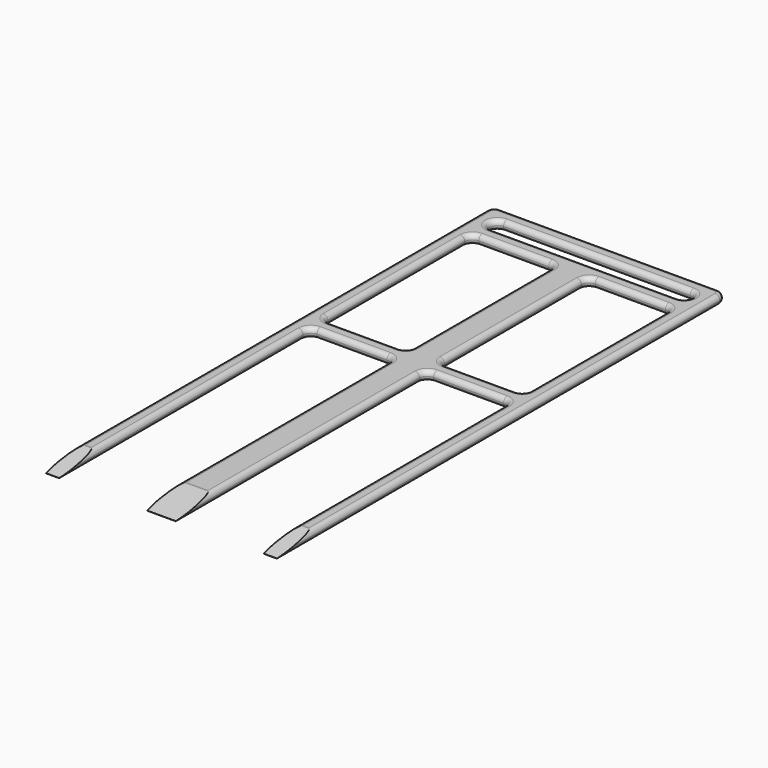
from build123d import *

# Parameters (mm, degrees)
F1_DEPTH     = 3
F2_SIZE2     = 14.178204549
F2_SIZE      = 2.5
F2_2_SIZE2   = 14.178204549
F2_2_SIZE    = 2.5
F2_3_SIZE2   = 14.178204549
F2_3_SIZE    = 2.5
F3_T1_DEPTH  = 174.571795451
F3_T3_DEPTH  = 5.6561649764
F3_T5_DEPTH  = 94.571795451
F3_T7_DEPTH  = 70
F3_T9_DEPTH  = 22.5
F3_T11_DEPTH = 5.6561649764
F3_T13_DEPTH = 10.6561649764
F3_T15_DEPTH = 22.5
F3_T17_DEPTH = 55
F3_T19_DEPTH = 60
F3_T21_DEPTH = 181.25
F3_T23_DEPTH = 10.5901699437
F3_T25_DEPTH = 101.25
F3_T27_DEPTH = 15.5901699437
F3_T29_DEPTH = 10.5901699437
F3_T32_ANGLE = 90
F3_T34_ANGLE = 90
F3_T36_ANGLE = 90
F3_T38_ANGLE = 90
F3_T40_ANGLE = 90
F3_T42_ANGLE = 90
F3_T44_ANGLE = 90
F3_T46_ANGLE = 90
F3_T48_ANGLE = 90
F3_T50_ANGLE = 90
F3_T52_ANGLE = 180
F3_T54_ANGLE = 180
F3_T56_ANGLE = 90
F3_T58_ANGLE = 90
F3_T60_ANGLE = 90
F3_T62_ANGLE = 90
F3_T64_ANGLE = 90
F3_T66_ANGLE = 90
F3_T68_ANGLE = 90
F3_T70_ANGLE = 90
F3_T72_ANGLE = 90
F3_T74_ANGLE = 90
F3_T76_ANGLE = 90
F3_T78_ANGLE = 90
F3_T80_ANGLE = 90
F3_T82_ANGLE = 90
F3_T84_ANGLE = 180
F3_T86_ANGLE = 180
F3_T88_ANGLE = 90
F3_T90_ANGLE = 90
F3_T92_ANGLE = 90
F3_T94_ANGLE = 90


# Not quite as in the source:
# - a fillet or chamfer that OpenCascade refuses, or shapes differently, is made with other operations: its cross-section is extruded or revolved along the edge and cut away or added


with BuildPart() as f1:
    # F0 (on Top) → F1 (new body)
    with BuildSketch(Plane.XY):
        with BuildLine():
            ThreePointArc((37.5, 87.5), (36.767766953, 89.267766953), (35, 90))
            Line((35, 90), (-35, 90))
            ThreePointArc((-35, 90), (-36.767766953, 89.267766953), (-37.5, 87.5))
            Line((-37.5, 87.5), (-37.5, -90))
            Line((-37.5, -90), (-32.5, -90))
            Line((-32.5, -90), (-32.5, 7.5))
            ThreePointArc((-32.5, 7.5), (-31.767766953, 9.267766953), (-30, 10))
            Line((-30, 10), (-7.5, 10))
            ThreePointArc((-7.5, 10), (-5.732233047, 9.267766953), (-5, 7.5))
            Line((-5, 7.5), (-5, -90))
            Line((-5, -90), (5, -90))
            Line((5, -90), (5, 7.5))
            ThreePointArc((5, 7.5), (5.732233047, 9.267766953), (7.5, 10))
            Line((7.5, 10), (30, 10))
            ThreePointArc((30, 10), (31.767766953, 9.267766953), (32.5, 7.5))
            Line((32.5, 7.5), (32.5, -90))
            Line((32.5, -90), (37.5, -90))
            Line((37.5, -90), (37.5, 87.5))
        make_face()
        with BuildLine():
            ThreePointArc((-5, 17.5), (-5.732233047, 15.732233047), (-7.5, 15))
            Line((-7.5, 15), (-30, 15))
            ThreePointArc((-30, 15), (-31.767766953, 15.732233047), (-32.5, 17.5))
            Line((-32.5, 17.5), (-32.5, 72.5))
            ThreePointArc((-32.5, 72.5), (-31.767766953, 74.267766953), (-30, 75))
            Line((-30, 75), (-7.5, 75))
            ThreePointArc((-7.5, 75), (-5.732233047, 74.267766953), (-5, 72.5))
            Line((-5, 72.5), (-5, 17.5))
        make_face(mode=Mode.SUBTRACT)
        with BuildLine():
            ThreePointArc((32.5, 82.5), (31.767766953, 80.732233047), (30, 80))
            Line((30, 80), (-30, 80))
            ThreePointArc((-30, 80), (-31.767766953, 80.732233047), (-32.5, 82.5))
            ThreePointArc((-32.5, 82.5), (-31.767766953, 84.267766953), (-30, 85))
            Line((-30, 85), (30, 85))
            ThreePointArc((30, 85), (31.767766953, 84.267766953), (32.5, 82.5))
        make_face(mode=Mode.SUBTRACT)
        with BuildLine():
            ThreePointArc((32.5, 17.5), (31.767766953, 15.732233047), (30, 15))
            Line((30, 15), (7.5, 15))
            ThreePointArc((7.5, 15), (5.732233047, 15.732233047), (5, 17.5))
            Line((5, 17.5), (5, 72.5))
            ThreePointArc((5, 72.5), (5.732233047, 74.267766953), (7.5, 75))
            Line((7.5, 75), (30, 75))
            ThreePointArc((30, 75), (31.767766953, 74.267766953), (32.5, 72.5))
            Line((32.5, 72.5), (32.5, 17.5))
        make_face(mode=Mode.SUBTRACT)
    extrude(amount=F1_DEPTH)

    # F2
    f2_edges = [f1.edges().sort_by_distance(p)[0] for p in [
        (0, -90, 3),
    ]]
    f2_side = f1.faces().sort_by_distance((0, -90, 1.5))[0]
    chamfer(f2_edges, length=F2_SIZE, length2=F2_SIZE2, reference=f2_side)

    # F2#2
    f2_2_edges = [f1.edges().sort_by_distance(p)[0] for p in [
        (35, -90, 3),
    ]]
    f2_2_side = f1.faces().sort_by_distance((35, -90, 1.5))[0]
    chamfer(f2_2_edges, length=F2_2_SIZE, length2=F2_2_SIZE2, reference=f2_2_side)

    # F2#3
    f2_3_edges = [f1.edges().sort_by_distance(p)[0] for p in [
        (-35, -90, 3),
    ]]
    f2_3_side = f1.faces().sort_by_distance((-35, -90, 1.5))[0]
    chamfer(f2_3_edges, length=F2_3_SIZE, length2=F2_3_SIZE2, reference=f2_3_side)

    # F3: fillet of radius 1.5 on 76 edges, made by hand

    # F3_s2 → F3_t1 (cut)
    with BuildSketch(Plane.XZ.offset(-87.5)):
        with BuildLine():
            ThreePointArc((-36, 3), (-37.0606601718, 2.5606601718), (-37.5, 1.5))
            Line((-37.5, 1.5), (-37.53, 1.5))
            Line((-37.53, 1.5), (-37.53, 3.03))
            Line((-37.53, 3.03), (-36, 3.03))
            Line((-36, 3.03), (-36, 3))
        make_face()
        with BuildLine():
            ThreePointArc((36, 3), (37.0606601718, 2.5606601718), (37.5, 1.5))
            Line((37.5, 1.5), (37.53, 1.5))
            Line((37.53, 1.5), (37.53, 3.03))
            Line((37.53, 3.03), (36, 3.03))
            Line((36, 3.03), (36, 3))
        make_face()
    extrude(amount=F3_T1_DEPTH, mode=Mode.SUBTRACT)

    # F3_s4 → F3_t3 (cut)
    with BuildSketch(Plane.YZ.offset(-37.8280824882)):
        with BuildLine():
            ThreePointArc((-75.6905624557, 3), (-75.8212960698, 2.9942920471), (-75.9510347222, 2.9772116295))
            Line((-75.9510347222, 2.9772116295), (-75.9562441675, 3.0067558621))
            Line((-75.9562441675, 3.0067558621), (-75.8244201109, 3.03))
            Line((-75.8244201109, 3.03), (-75.6905624557, 3.03))
            Line((-75.6905624557, 3.03), (-75.6905624557, 3))
        make_face()
    extrude(amount=F3_T3_DEPTH, mode=Mode.SUBTRACT)

    # F3_s6 → F3_t5 (cut)
    with BuildSketch(Plane.XZ.offset(-7.5)):
        with BuildLine():
            ThreePointArc((-34, 3), (-32.9393398282, 2.5606601718), (-32.5, 1.5))
            Line((-32.5, 1.5), (-32.47, 1.5))
            Line((-32.47, 1.5), (-32.47, 3.03))
            Line((-32.47, 3.03), (-34, 3.03))
            Line((-34, 3.03), (-34, 3))
        make_face()
        with BuildLine():
            ThreePointArc((-3.5, 3), (-4.5606601718, 2.5606601718), (-5, 1.5))
            Line((-5, 1.5), (-5.03, 1.5))
            Line((-5.03, 1.5), (-5.03, 3.03))
            Line((-5.03, 3.03), (-3.5, 3.03))
            Line((-3.5, 3.03), (-3.5, 3))
        make_face()
        with BuildLine():
            ThreePointArc((34, 3), (32.9393398282, 2.5606601718), (32.5, 1.5))
            Line((32.5, 1.5), (32.47, 1.5))
            Line((32.47, 1.5), (32.47, 3.03))
            Line((32.47, 3.03), (34, 3.03))
            Line((34, 3.03), (34, 3))
        make_face()
        with BuildLine():
            ThreePointArc((3.5, 3), (4.5606601718, 2.5606601718), (5, 1.5))
            Line((5, 1.5), (5.03, 1.5))
            Line((5.03, 1.5), (5.03, 3.03))
            Line((5.03, 3.03), (3.5, 3.03))
            Line((3.5, 3.03), (3.5, 3))
        make_face()
    extrude(amount=F3_T5_DEPTH, mode=Mode.SUBTRACT)

    # F3_s8 → F3_t7 (cut)
    with BuildSketch(Plane.YZ.offset(-35)):
        with BuildLine():
            ThreePointArc((88.5, 3), (89.5606601718, 2.5606601718), (90, 1.5))
            Line((90, 1.5), (90.03, 1.5))
            Line((90.03, 1.5), (90.03, 3.03))
            Line((90.03, 3.03), (88.5, 3.03))
            Line((88.5, 3.03), (88.5, 3))
        make_face()
        with BuildLine():
            ThreePointArc((90, 1.5), (89.5606601718, 0.4393398282), (88.5, 0))
            Line((88.5, 0), (88.5, -0.03))
            Line((88.5, -0.03), (90.03, -0.03))
            Line((90.03, -0.03), (90.03, 1.5))
            Line((90.03, 1.5), (90, 1.5))
        make_face()
    extrude(amount=F3_T7_DEPTH, mode=Mode.SUBTRACT)

    # F3_s10 → F3_t9 (cut)
    with BuildSketch(Plane.YZ.offset(-30)):
        with BuildLine():
            ThreePointArc((11.5, 3), (10.4393398282, 2.5606601718), (10, 1.5))
            Line((10, 1.5), (9.97, 1.5))
            Line((9.97, 1.5), (9.97, 3.03))
            Line((9.97, 3.03), (11.5, 3.03))
            Line((11.5, 3.03), (11.5, 3))
        make_face()
        with BuildLine():
            ThreePointArc((13.5, 3), (14.5606601718, 2.5606601718), (15, 1.5))
            Line((15, 1.5), (15.03, 1.5))
            Line((15.03, 1.5), (15.03, 3.03))
            Line((15.03, 3.03), (13.5, 3.03))
            Line((13.5, 3.03), (13.5, 3))
        make_face()
        with BuildLine():
            ThreePointArc((76.5, 3), (75.4393398282, 2.5606601718), (75, 1.5))
            Line((75, 1.5), (74.97, 1.5))
            Line((74.97, 1.5), (74.97, 3.03))
            Line((74.97, 3.03), (76.5, 3.03))
            Line((76.5, 3.03), (76.5, 3))
        make_face()
        with BuildLine():
            ThreePointArc((10, 1.5), (10.4393398282, 0.4393398282), (11.5, 0))
            Line((11.5, 0), (11.5, -0.03))
            Line((11.5, -0.03), (9.97, -0.03))
            Line((9.97, -0.03), (9.97, 1.5))
            Line((9.97, 1.5), (10, 1.5))
        make_face()
        with BuildLine():
            ThreePointArc((15, 1.5), (14.5606601718, 0.4393398282), (13.5, 0))
            Line((13.5, 0), (13.5, -0.03))
            Line((13.5, -0.03), (15.03, -0.03))
            Line((15.03, -0.03), (15.03, 1.5))
            Line((15.03, 1.5), (15, 1.5))
        make_face()
        with BuildLine():
            ThreePointArc((75, 1.5), (75.4393398282, 0.4393398282), (76.5, 0))
            Line((76.5, 0), (76.5, -0.03))
            Line((76.5, -0.03), (74.97, -0.03))
            Line((74.97, -0.03), (74.97, 1.5))
            Line((74.97, 1.5), (75, 1.5))
        make_face()
    extrude(amount=F3_T9_DEPTH, mode=Mode.SUBTRACT)

    # F3_s12 → F3_t11 (cut)
    with BuildSketch(Plane.YZ.offset(32.1719175118)):
        with BuildLine():
            ThreePointArc((-75.6905624557, 3), (-75.8212960698, 2.9942920471), (-75.9510347222, 2.9772116295))
            Line((-75.9510347222, 2.9772116295), (-75.9562441675, 3.0067558621))
            Line((-75.9562441675, 3.0067558621), (-75.8244201109, 3.03))
            Line((-75.8244201109, 3.03), (-75.6905624557, 3.03))
            Line((-75.6905624557, 3.03), (-75.6905624557, 3))
        make_face()
    extrude(amount=F3_T11_DEPTH, mode=Mode.SUBTRACT)

    # F3_s14 → F3_t13 (cut)
    with BuildSketch(Plane.YZ.offset(-5.3280824882)):
        with BuildLine():
            ThreePointArc((-75.6905624557, 3), (-75.8212960698, 2.9942920471), (-75.9510347222, 2.9772116295))
            Line((-75.9510347222, 2.9772116295), (-75.9562441675, 3.0067558621))
            Line((-75.9562441675, 3.0067558621), (-75.8244201109, 3.03))
            Line((-75.8244201109, 3.03), (-75.6905624557, 3.03))
            Line((-75.6905624557, 3.03), (-75.6905624557, 3))
        make_face()
    extrude(amount=F3_T13_DEPTH, mode=Mode.SUBTRACT)

    # F3_s16 → F3_t15 (cut)
    with BuildSketch(Plane.YZ.offset(7.5)):
        with BuildLine():
            ThreePointArc((11.5, 3), (10.4393398282, 2.5606601718), (10, 1.5))
            Line((10, 1.5), (9.97, 1.5))
            Line((9.97, 1.5), (9.97, 3.03))
            Line((9.97, 3.03), (11.5, 3.03))
            Line((11.5, 3.03), (11.5, 3))
        make_face()
        with BuildLine():
            ThreePointArc((13.5, 3), (14.5606601718, 2.5606601718), (15, 1.5))
            Line((15, 1.5), (15.03, 1.5))
            Line((15.03, 1.5), (15.03, 3.03))
            Line((15.03, 3.03), (13.5, 3.03))
            Line((13.5, 3.03), (13.5, 3))
        make_face()
        with BuildLine():
            ThreePointArc((76.5, 3), (75.4393398282, 2.5606601718), (75, 1.5))
            Line((75, 1.5), (74.97, 1.5))
            Line((74.97, 1.5), (74.97, 3.03))
            Line((74.97, 3.03), (76.5, 3.03))
            Line((76.5, 3.03), (76.5, 3))
        make_face()
        with BuildLine():
            ThreePointArc((10, 1.5), (10.4393398282, 0.4393398282), (11.5, 0))
            Line((11.5, 0), (11.5, -0.03))
            Line((11.5, -0.03), (9.97, -0.03))
            Line((9.97, -0.03), (9.97, 1.5))
            Line((9.97, 1.5), (10, 1.5))
        make_face()
        with BuildLine():
            ThreePointArc((15, 1.5), (14.5606601718, 0.4393398282), (13.5, 0))
            Line((13.5, 0), (13.5, -0.03))
            Line((13.5, -0.03), (15.03, -0.03))
            Line((15.03, -0.03), (15.03, 1.5))
            Line((15.03, 1.5), (15, 1.5))
        make_face()
        with BuildLine():
            ThreePointArc((75, 1.5), (75.4393398282, 0.4393398282), (76.5, 0))
            Line((76.5, 0), (76.5, -0.03))
            Line((76.5, -0.03), (74.97, -0.03))
            Line((74.97, -0.03), (74.97, 1.5))
            Line((74.97, 1.5), (75, 1.5))
        make_face()
    extrude(amount=F3_T15_DEPTH, mode=Mode.SUBTRACT)

    # F3_s18 → F3_t17 (cut)
    with BuildSketch(Plane.XZ.offset(-72.5)):
        with BuildLine():
            ThreePointArc((-34, 3), (-32.9393398282, 2.5606601718), (-32.5, 1.5))
            Line((-32.5, 1.5), (-32.47, 1.5))
            Line((-32.47, 1.5), (-32.47, 3.03))
            Line((-32.47, 3.03), (-34, 3.03))
            Line((-34, 3.03), (-34, 3))
        make_face()
        with BuildLine():
            ThreePointArc((-3.5, 3), (-4.5606601718, 2.5606601718), (-5, 1.5))
            Line((-5, 1.5), (-5.03, 1.5))
            Line((-5.03, 1.5), (-5.03, 3.03))
            Line((-5.03, 3.03), (-3.5, 3.03))
            Line((-3.5, 3.03), (-3.5, 3))
        make_face()
        with BuildLine():
            ThreePointArc((34, 3), (32.9393398282, 2.5606601718), (32.5, 1.5))
            Line((32.5, 1.5), (32.47, 1.5))
            Line((32.47, 1.5), (32.47, 3.03))
            Line((32.47, 3.03), (34, 3.03))
            Line((34, 3.03), (34, 3))
        make_face()
        with BuildLine():
            ThreePointArc((3.5, 3), (4.5606601718, 2.5606601718), (5, 1.5))
            Line((5, 1.5), (5.03, 1.5))
            Line((5.03, 1.5), (5.03, 3.03))
            Line((5.03, 3.03), (3.5, 3.03))
            Line((3.5, 3.03), (3.5, 3))
        make_face()
        with BuildLine():
            ThreePointArc((-32.5, 1.5), (-32.9393398282, 0.4393398282), (-34, 0))
            Line((-34, 0), (-34, -0.03))
            Line((-34, -0.03), (-32.47, -0.03))
            Line((-32.47, -0.03), (-32.47, 1.5))
            Line((-32.47, 1.5), (-32.5, 1.5))
        make_face()
        with BuildLine():
            ThreePointArc((-5, 1.5), (-4.5606601718, 0.4393398282), (-3.5, 0))
            Line((-3.5, 0), (-3.5, -0.03))
            Line((-3.5, -0.03), (-5.03, -0.03))
            Line((-5.03, -0.03), (-5.03, 1.5))
            Line((-5.03, 1.5), (-5, 1.5))
        make_face()
        with BuildLine():
            ThreePointArc((32.5, 1.5), (32.9393398282, 0.4393398282), (34, 0))
            Line((34, 0), (34, -0.03))
            Line((34, -0.03), (32.47, -0.03))
            Line((32.47, -0.03), (32.47, 1.5))
            Line((32.47, 1.5), (32.5, 1.5))
        make_face()
        with BuildLine():
            ThreePointArc((5, 1.5), (4.5606601718, 0.4393398282), (3.5, 0))
            Line((3.5, 0), (3.5, -0.03))
            Line((3.5, -0.03), (5.03, -0.03))
            Line((5.03, -0.03), (5.03, 1.5))
            Line((5.03, 1.5), (5, 1.5))
        make_face()
    extrude(amount=F3_T17_DEPTH, mode=Mode.SUBTRACT)

    # F3_s20 → F3_t19 (cut)
    with BuildSketch(Plane.YZ.offset(-30)):
        with BuildLine():
            ThreePointArc((78.5, 3), (79.5606601718, 2.5606601718), (80, 1.5))
            Line((80, 1.5), (80.03, 1.5))
            Line((80.03, 1.5), (80.03, 3.03))
            Line((80.03, 3.03), (78.5, 3.03))
            Line((78.5, 3.03), (78.5, 3))
        make_face()
        with BuildLine():
            ThreePointArc((86.5, 3), (85.4393398282, 2.5606601718), (85, 1.5))
            Line((85, 1.5), (84.97, 1.5))
            Line((84.97, 1.5), (84.97, 3.03))
            Line((84.97, 3.03), (86.5, 3.03))
            Line((86.5, 3.03), (86.5, 3))
        make_face()
        with BuildLine():
            ThreePointArc((80, 1.5), (79.5606601718, 0.4393398282), (78.5, 0))
            Line((78.5, 0), (78.5, -0.03))
            Line((78.5, -0.03), (80.03, -0.03))
            Line((80.03, -0.03), (80.03, 1.5))
            Line((80.03, 1.5), (80, 1.5))
        make_face()
        with BuildLine():
            ThreePointArc((85, 1.5), (85.4393398282, 0.4393398282), (86.5, 0))
            Line((86.5, 0), (86.5, -0.03))
            Line((86.5, -0.03), (84.97, -0.03))
            Line((84.97, -0.03), (84.97, 1.5))
            Line((84.97, 1.5), (85, 1.5))
        make_face()
    extrude(amount=F3_T19_DEPTH, mode=Mode.SUBTRACT)

    # F3_s22 → F3_t21 (cut)
    with BuildSketch(Plane.XZ.offset(-87.5)):
        with BuildLine():
            ThreePointArc((-37.5, 1.5), (-37.0606601718, 0.4393398282), (-36, 0))
            Line((-36, 0), (-36, -0.03))
            Line((-36, -0.03), (-37.53, -0.03))
            Line((-37.53, -0.03), (-37.53, 1.5))
            Line((-37.53, 1.5), (-37.5, 1.5))
        make_face()
        with BuildLine():
            ThreePointArc((37.5, 1.5), (37.0606601718, 0.4393398282), (36, 0))
            Line((36, 0), (36, -0.03))
            Line((36, -0.03), (37.53, -0.03))
            Line((37.53, -0.03), (37.53, 1.5))
            Line((37.53, 1.5), (37.5, 1.5))
        make_face()
    extrude(amount=F3_T21_DEPTH, mode=Mode.SUBTRACT)

    # F3_s24 → F3_t23 (cut)
    with BuildSketch(Plane.YZ.offset(-40.2950849719)):
        with BuildLine():
            ThreePointArc((-90, 0.5), (-89.4943384469, 0.1306936062), (-88.8819660113, 0))
            Line((-88.8819660113, 0), (-88.8819660113, -0.03))
            Line((-88.8819660113, -0.03), (-90, -0.03))
            Line((-90, -0.03), (-90.03, 0))
            ThreePointArc((-90.03, 0), (-90.03, 0.25), (-90.0223606798, 0.48))
            Line((-90.0223606798, 0.48), (-90, 0.5))
        make_face()
    extrude(amount=F3_T23_DEPTH, mode=Mode.SUBTRACT)

    # F3_s26 → F3_t25 (cut)
    with BuildSketch(Plane.XZ.offset(-7.5)):
        with BuildLine():
            ThreePointArc((-32.5, 1.5), (-32.9393398282, 0.4393398282), (-34, 0))
            Line((-34, 0), (-34, -0.03))
            Line((-34, -0.03), (-32.47, -0.03))
            Line((-32.47, -0.03), (-32.47, 1.5))
            Line((-32.47, 1.5), (-32.5, 1.5))
        make_face()
        with BuildLine():
            ThreePointArc((-5, 1.5), (-4.5606601718, 0.4393398282), (-3.5, 0))
            Line((-3.5, 0), (-3.5, -0.03))
            Line((-3.5, -0.03), (-5.03, -0.03))
            Line((-5.03, -0.03), (-5.03, 1.5))
            Line((-5.03, 1.5), (-5, 1.5))
        make_face()
        with BuildLine():
            ThreePointArc((5, 1.5), (4.5606601718, 0.4393398282), (3.5, 0))
            Line((3.5, 0), (3.5, -0.03))
            Line((3.5, -0.03), (5.03, -0.03))
            Line((5.03, -0.03), (5.03, 1.5))
            Line((5.03, 1.5), (5, 1.5))
        make_face()
        with BuildLine():
            ThreePointArc((32.5, 1.5), (32.9393398282, 0.4393398282), (34, 0))
            Line((34, 0), (34, -0.03))
            Line((34, -0.03), (32.47, -0.03))
            Line((32.47, -0.03), (32.47, 1.5))
            Line((32.47, 1.5), (32.5, 1.5))
        make_face()
    extrude(amount=F3_T25_DEPTH, mode=Mode.SUBTRACT)

    # F3_s28 → F3_t27 (cut)
    with BuildSketch(Plane.YZ.offset(-7.7950849719)):
        with BuildLine():
            ThreePointArc((-88.8819660113, 0), (-89.4943384469, 0.1306936062), (-90, 0.5))
            Line((-90, 0.5), (-90.0223606798, 0.48))
            ThreePointArc((-90.0223606798, 0.48), (-90.03, 0.25), (-90.03, 0))
            Line((-90.03, 0), (-90, -0.03))
            Line((-90, -0.03), (-88.8819660113, -0.03))
            Line((-88.8819660113, -0.03), (-88.8819660113, 0))
        make_face()
    extrude(amount=F3_T27_DEPTH, mode=Mode.SUBTRACT)

    # F3_s30 → F3_t29 (cut)
    with BuildSketch(Plane.YZ.offset(29.7049150281)):
        with BuildLine():
            ThreePointArc((-88.8819660113, 0), (-89.4943384469, 0.1306936062), (-90, 0.5))
            Line((-90, 0.5), (-90.0223606798, 0.48))
            ThreePointArc((-90.0223606798, 0.48), (-90.03, 0.25), (-90.03, 0))
            Line((-90.03, 0), (-90, -0.03))
            Line((-90, -0.03), (-88.8819660113, -0.03))
            Line((-88.8819660113, -0.03), (-88.8819660113, 0))
        make_face()
    extrude(amount=F3_T29_DEPTH, mode=Mode.SUBTRACT)

    # F3_s31 → F3_t32 (revolve, cut)
    with BuildSketch(Plane.YZ.offset(-35)):
        with BuildLine():
            ThreePointArc((88.5, 3), (89.5606601718, 2.5606601718), (90, 1.5))
            Line((90, 1.5), (90.03, 1.5))
            Line((90.03, 1.5), (90.03, 3.03))
            Line((90.03, 3.03), (88.5, 3.03))
            Line((88.5, 3.03), (88.5, 3))
        make_face()
    revolve(axis=Axis((-35, 87.5, 3), (0, 0, 1)), revolution_arc=F3_T32_ANGLE, mode=Mode.SUBTRACT)

    # F3_s33 → F3_t34 (revolve, cut)
    with BuildSketch(Plane.XZ.offset(-7.5)):
        with BuildLine():
            ThreePointArc((-34, 3), (-32.9393398282, 2.5606601718), (-32.5, 1.5))
            Line((-32.5, 1.5), (-32.47, 1.5))
            Line((-32.47, 1.5), (-32.47, 3.03))
            Line((-32.47, 3.03), (-34, 3.03))
            Line((-34, 3.03), (-34, 3))
        make_face()
    revolve(axis=Axis((-30, 7.5, 3), (0, 0, -1)), revolution_arc=F3_T34_ANGLE, mode=Mode.SUBTRACT)

    # F3_s35 → F3_t36 (revolve, cut)
    with BuildSketch(Plane.XZ.offset(-87.5)):
        with BuildLine():
            ThreePointArc((36, 3), (37.0606601718, 2.5606601718), (37.5, 1.5))
            Line((37.5, 1.5), (37.53, 1.5))
            Line((37.53, 1.5), (37.53, 3.03))
            Line((37.53, 3.03), (36, 3.03))
            Line((36, 3.03), (36, 3))
        make_face()
    revolve(axis=Axis((35, 87.5, 3), (0, 0, 1)), revolution_arc=F3_T36_ANGLE, mode=Mode.SUBTRACT)

    # F3_s37 → F3_t38 (revolve, cut)
    with BuildSketch(Plane.YZ.offset(-7.5)):
        with BuildLine():
            ThreePointArc((11.5, 3), (10.4393398282, 2.5606601718), (10, 1.5))
            Line((10, 1.5), (9.97, 1.5))
            Line((9.97, 1.5), (9.97, 3.03))
            Line((9.97, 3.03), (11.5, 3.03))
            Line((11.5, 3.03), (11.5, 3))
        make_face()
    revolve(axis=Axis((-7.5, 7.5, 3), (0, 0, -1)), revolution_arc=F3_T38_ANGLE, mode=Mode.SUBTRACT)

    # F3_s39 → F3_t40 (revolve, cut)
    with BuildSketch(Plane.YZ.offset(30)):
        with BuildLine():
            ThreePointArc((11.5, 3), (10.4393398282, 2.5606601718), (10, 1.5))
            Line((10, 1.5), (9.97, 1.5))
            Line((9.97, 1.5), (9.97, 3.03))
            Line((9.97, 3.03), (11.5, 3.03))
            Line((11.5, 3.03), (11.5, 3))
        make_face()
    revolve(axis=Axis((30, 7.5, 3), (0, 0, -1)), revolution_arc=F3_T40_ANGLE, mode=Mode.SUBTRACT)

    # F3_s41 → F3_t42 (revolve, cut)
    with BuildSketch(Plane.XZ.offset(-7.5)):
        with BuildLine():
            ThreePointArc((3.5, 3), (4.5606601718, 2.5606601718), (5, 1.5))
            Line((5, 1.5), (5.03, 1.5))
            Line((5.03, 1.5), (5.03, 3.03))
            Line((5.03, 3.03), (3.5, 3.03))
            Line((3.5, 3.03), (3.5, 3))
        make_face()
    revolve(axis=Axis((7.5, 7.5, 3), (0, 0, -1)), revolution_arc=F3_T42_ANGLE, mode=Mode.SUBTRACT)

    # F3_s43 → F3_t44 (revolve, cut)
    with BuildSketch(Plane.XZ.offset(-17.5)):
        with BuildLine():
            ThreePointArc((-3.5, 3), (-4.5606601718, 2.5606601718), (-5, 1.5))
            Line((-5, 1.5), (-5.03, 1.5))
            Line((-5.03, 1.5), (-5.03, 3.03))
            Line((-5.03, 3.03), (-3.5, 3.03))
            Line((-3.5, 3.03), (-3.5, 3))
        make_face()
    revolve(axis=Axis((-7.5, 17.5, 3), (0, 0, -1)), revolution_arc=F3_T44_ANGLE, mode=Mode.SUBTRACT)

    # F3_s45 → F3_t46 (revolve, cut)
    with BuildSketch(Plane.YZ.offset(-30)):
        with BuildLine():
            ThreePointArc((13.5, 3), (14.5606601718, 2.5606601718), (15, 1.5))
            Line((15, 1.5), (15.03, 1.5))
            Line((15.03, 1.5), (15.03, 3.03))
            Line((15.03, 3.03), (13.5, 3.03))
            Line((13.5, 3.03), (13.5, 3))
        make_face()
    revolve(axis=Axis((-30, 17.5, 3), (0, 0, -1)), revolution_arc=F3_T46_ANGLE, mode=Mode.SUBTRACT)

    # F3_s47 → F3_t48 (revolve, cut)
    with BuildSketch(Plane.XZ.offset(-72.5)):
        with BuildLine():
            ThreePointArc((-34, 3), (-32.9393398282, 2.5606601718), (-32.5, 1.5))
            Line((-32.5, 1.5), (-32.47, 1.5))
            Line((-32.47, 1.5), (-32.47, 3.03))
            Line((-32.47, 3.03), (-34, 3.03))
            Line((-34, 3.03), (-34, 3))
        make_face()
    revolve(axis=Axis((-30, 72.5, 3), (0, 0, -1)), revolution_arc=F3_T48_ANGLE, mode=Mode.SUBTRACT)

    # F3_s49 → F3_t50 (revolve, cut)
    with BuildSketch(Plane.YZ.offset(-7.5)):
        with BuildLine():
            ThreePointArc((76.5, 3), (75.4393398282, 2.5606601718), (75, 1.5))
            Line((75, 1.5), (74.97, 1.5))
            Line((74.97, 1.5), (74.97, 3.03))
            Line((74.97, 3.03), (76.5, 3.03))
            Line((76.5, 3.03), (76.5, 3))
        make_face()
    revolve(axis=Axis((-7.5, 72.5, 3), (0, 0, -1)), revolution_arc=F3_T50_ANGLE, mode=Mode.SUBTRACT)

    # F3_s51 → F3_t52 (revolve, cut)
    with BuildSketch(Plane.YZ.offset(30)):
        with BuildLine():
            ThreePointArc((78.5, 3), (79.5606601718, 2.5606601718), (80, 1.5))
            Line((80, 1.5), (80.03, 1.5))
            Line((80.03, 1.5), (80.03, 3.03))
            Line((80.03, 3.03), (78.5, 3.03))
            Line((78.5, 3.03), (78.5, 3))
        make_face()
    revolve(axis=Axis((30, 82.5, 3), (0, 0, 1)), revolution_arc=F3_T52_ANGLE, mode=Mode.SUBTRACT)

    # F3_s53 → F3_t54 (revolve, cut)
    with BuildSketch(Plane.YZ.offset(-30)):
        with BuildLine():
            ThreePointArc((86.5, 3), (85.4393398282, 2.5606601718), (85, 1.5))
            Line((85, 1.5), (84.97, 1.5))
            Line((84.97, 1.5), (84.97, 3.03))
            Line((84.97, 3.03), (86.5, 3.03))
            Line((86.5, 3.03), (86.5, 3))
        make_face()
    revolve(axis=Axis((-30, 82.5, 3), (0, 0, 1)), revolution_arc=F3_T54_ANGLE, mode=Mode.SUBTRACT)

    # F3_s55 → F3_t56 (revolve, cut)
    with BuildSketch(Plane.XZ.offset(-17.5)):
        with BuildLine():
            ThreePointArc((34, 3), (32.9393398282, 2.5606601718), (32.5, 1.5))
            Line((32.5, 1.5), (32.47, 1.5))
            Line((32.47, 1.5), (32.47, 3.03))
            Line((32.47, 3.03), (34, 3.03))
            Line((34, 3.03), (34, 3))
        make_face()
    revolve(axis=Axis((30, 17.5, 3), (0, 0, -1)), revolution_arc=F3_T56_ANGLE, mode=Mode.SUBTRACT)

    # F3_s57 → F3_t58 (revolve, cut)
    with BuildSketch(Plane.YZ.offset(7.5)):
        with BuildLine():
            ThreePointArc((13.5, 3), (14.5606601718, 2.5606601718), (15, 1.5))
            Line((15, 1.5), (15.03, 1.5))
            Line((15.03, 1.5), (15.03, 3.03))
            Line((15.03, 3.03), (13.5, 3.03))
            Line((13.5, 3.03), (13.5, 3))
        make_face()
    revolve(axis=Axis((7.5, 17.5, 3), (0, 0, -1)), revolution_arc=F3_T58_ANGLE, mode=Mode.SUBTRACT)

    # F3_s59 → F3_t60 (revolve, cut)
    with BuildSketch(Plane.XZ.offset(-72.5)):
        with BuildLine():
            ThreePointArc((3.5, 3), (4.5606601718, 2.5606601718), (5, 1.5))
            Line((5, 1.5), (5.03, 1.5))
            Line((5.03, 1.5), (5.03, 3.03))
            Line((5.03, 3.03), (3.5, 3.03))
            Line((3.5, 3.03), (3.5, 3))
        make_face()
    revolve(axis=Axis((7.5, 72.5, 3), (0, 0, -1)), revolution_arc=F3_T60_ANGLE, mode=Mode.SUBTRACT)

    # F3_s61 → F3_t62 (revolve, cut)
    with BuildSketch(Plane.YZ.offset(30)):
        with BuildLine():
            ThreePointArc((76.5, 3), (75.4393398282, 2.5606601718), (75, 1.5))
            Line((75, 1.5), (74.97, 1.5))
            Line((74.97, 1.5), (74.97, 3.03))
            Line((74.97, 3.03), (76.5, 3.03))
            Line((76.5, 3.03), (76.5, 3))
        make_face()
    revolve(axis=Axis((30, 72.5, 3), (0, 0, -1)), revolution_arc=F3_T62_ANGLE, mode=Mode.SUBTRACT)

    # F3_s63 → F3_t64 (revolve, cut)
    with BuildSketch(Plane.XZ.offset(-87.5)):
        with BuildLine():
            ThreePointArc((37.5, 1.5), (37.0606601718, 0.4393398282), (36, 0))
            Line((36, 0), (36, -0.03))
            Line((36, -0.03), (37.53, -0.03))
            Line((37.53, -0.03), (37.53, 1.5))
            Line((37.53, 1.5), (37.5, 1.5))
        make_face()
    revolve(axis=Axis((35, 87.5, 0), (0, 0, 1)), revolution_arc=F3_T64_ANGLE, mode=Mode.SUBTRACT)

    # F3_s65 → F3_t66 (revolve, cut)
    with BuildSketch(Plane.YZ.offset(-35)):
        with BuildLine():
            ThreePointArc((90, 1.5), (89.5606601718, 0.4393398282), (88.5, 0))
            Line((88.5, 0), (88.5, -0.03))
            Line((88.5, -0.03), (90.03, -0.03))
            Line((90.03, -0.03), (90.03, 1.5))
            Line((90.03, 1.5), (90, 1.5))
        make_face()
    revolve(axis=Axis((-35, 87.5, 0), (0, 0, 1)), revolution_arc=F3_T66_ANGLE, mode=Mode.SUBTRACT)

    # F3_s67 → F3_t68 (revolve, cut)
    with BuildSketch(Plane.XZ.offset(-7.5)):
        with BuildLine():
            ThreePointArc((-32.5, 1.5), (-32.9393398282, 0.4393398282), (-34, 0))
            Line((-34, 0), (-34, -0.03))
            Line((-34, -0.03), (-32.47, -0.03))
            Line((-32.47, -0.03), (-32.47, 1.5))
            Line((-32.47, 1.5), (-32.5, 1.5))
        make_face()
    revolve(axis=Axis((-30, 7.5, 0), (0, 0, -1)), revolution_arc=F3_T68_ANGLE, mode=Mode.SUBTRACT)

    # F3_s69 → F3_t70 (revolve, cut)
    with BuildSketch(Plane.YZ.offset(-7.5)):
        with BuildLine():
            ThreePointArc((10, 1.5), (10.4393398282, 0.4393398282), (11.5, 0))
            Line((11.5, 0), (11.5, -0.03))
            Line((11.5, -0.03), (9.97, -0.03))
            Line((9.97, -0.03), (9.97, 1.5))
            Line((9.97, 1.5), (10, 1.5))
        make_face()
    revolve(axis=Axis((-7.5, 7.5, 0), (0, 0, -1)), revolution_arc=F3_T70_ANGLE, mode=Mode.SUBTRACT)

    # F3_s71 → F3_t72 (revolve, cut)
    with BuildSketch(Plane.XZ.offset(-7.5)):
        with BuildLine():
            ThreePointArc((5, 1.5), (4.5606601718, 0.4393398282), (3.5, 0))
            Line((3.5, 0), (3.5, -0.03))
            Line((3.5, -0.03), (5.03, -0.03))
            Line((5.03, -0.03), (5.03, 1.5))
            Line((5.03, 1.5), (5, 1.5))
        make_face()
    revolve(axis=Axis((7.5, 7.5, 0), (0, 0, -1)), revolution_arc=F3_T72_ANGLE, mode=Mode.SUBTRACT)

    # F3_s73 → F3_t74 (revolve, cut)
    with BuildSketch(Plane.YZ.offset(30)):
        with BuildLine():
            ThreePointArc((10, 1.5), (10.4393398282, 0.4393398282), (11.5, 0))
            Line((11.5, 0), (11.5, -0.03))
            Line((11.5, -0.03), (9.97, -0.03))
            Line((9.97, -0.03), (9.97, 1.5))
            Line((9.97, 1.5), (10, 1.5))
        make_face()
    revolve(axis=Axis((30, 7.5, 0), (0, 0, -1)), revolution_arc=F3_T74_ANGLE, mode=Mode.SUBTRACT)

    # F3_s75 → F3_t76 (revolve, cut)
    with BuildSketch(Plane.XZ.offset(-17.5)):
        with BuildLine():
            ThreePointArc((-5, 1.5), (-4.5606601718, 0.4393398282), (-3.5, 0))
            Line((-3.5, 0), (-3.5, -0.03))
            Line((-3.5, -0.03), (-5.03, -0.03))
            Line((-5.03, -0.03), (-5.03, 1.5))
            Line((-5.03, 1.5), (-5, 1.5))
        make_face()
    revolve(axis=Axis((-7.5, 17.5, 0), (0, 0, -1)), revolution_arc=F3_T76_ANGLE, mode=Mode.SUBTRACT)

    # F3_s77 → F3_t78 (revolve, cut)
    with BuildSketch(Plane.YZ.offset(-30)):
        with BuildLine():
            ThreePointArc((15, 1.5), (14.5606601718, 0.4393398282), (13.5, 0))
            Line((13.5, 0), (13.5, -0.03))
            Line((13.5, -0.03), (15.03, -0.03))
            Line((15.03, -0.03), (15.03, 1.5))
            Line((15.03, 1.5), (15, 1.5))
        make_face()
    revolve(axis=Axis((-30, 17.5, 0), (0, 0, -1)), revolution_arc=F3_T78_ANGLE, mode=Mode.SUBTRACT)

    # F3_s79 → F3_t80 (revolve, cut)
    with BuildSketch(Plane.XZ.offset(-72.5)):
        with BuildLine():
            ThreePointArc((-32.5, 1.5), (-32.9393398282, 0.4393398282), (-34, 0))
            Line((-34, 0), (-34, -0.03))
            Line((-34, -0.03), (-32.47, -0.03))
            Line((-32.47, -0.03), (-32.47, 1.5))
            Line((-32.47, 1.5), (-32.5, 1.5))
        make_face()
    revolve(axis=Axis((-30, 72.5, 0), (0, 0, -1)), revolution_arc=F3_T80_ANGLE, mode=Mode.SUBTRACT)

    # F3_s81 → F3_t82 (revolve, cut)
    with BuildSketch(Plane.YZ.offset(-7.5)):
        with BuildLine():
            ThreePointArc((75, 1.5), (75.4393398282, 0.4393398282), (76.5, 0))
            Line((76.5, 0), (76.5, -0.03))
            Line((76.5, -0.03), (74.97, -0.03))
            Line((74.97, -0.03), (74.97, 1.5))
            Line((74.97, 1.5), (75, 1.5))
        make_face()
    revolve(axis=Axis((-7.5, 72.5, 0), (0, 0, -1)), revolution_arc=F3_T82_ANGLE, mode=Mode.SUBTRACT)

    # F3_s83 → F3_t84 (revolve, cut)
    with BuildSketch(Plane.YZ.offset(-30)):
        with BuildLine():
            ThreePointArc((80, 1.5), (79.5606601718, 0.4393398282), (78.5, 0))
            Line((78.5, 0), (78.5, -0.03))
            Line((78.5, -0.03), (80.03, -0.03))
            Line((80.03, -0.03), (80.03, 1.5))
            Line((80.03, 1.5), (80, 1.5))
        make_face()
    revolve(axis=Axis((-30, 82.5, 0), (0, 0, -1)), revolution_arc=F3_T84_ANGLE, mode=Mode.SUBTRACT)

    # F3_s85 → F3_t86 (revolve, cut)
    with BuildSketch(Plane.YZ.offset(30)):
        with BuildLine():
            ThreePointArc((85, 1.5), (85.4393398282, 0.4393398282), (86.5, 0))
            Line((86.5, 0), (86.5, -0.03))
            Line((86.5, -0.03), (84.97, -0.03))
            Line((84.97, -0.03), (84.97, 1.5))
            Line((84.97, 1.5), (85, 1.5))
        make_face()
    revolve(axis=Axis((30, 82.5, 0), (0, 0, -1)), revolution_arc=F3_T86_ANGLE, mode=Mode.SUBTRACT)

    # F3_s87 → F3_t88 (revolve, cut)
    with BuildSketch(Plane.XZ.offset(-17.5)):
        with BuildLine():
            ThreePointArc((32.5, 1.5), (32.9393398282, 0.4393398282), (34, 0))
            Line((34, 0), (34, -0.03))
            Line((34, -0.03), (32.47, -0.03))
            Line((32.47, -0.03), (32.47, 1.5))
            Line((32.47, 1.5), (32.5, 1.5))
        make_face()
    revolve(axis=Axis((30, 17.5, 0), (0, 0, -1)), revolution_arc=F3_T88_ANGLE, mode=Mode.SUBTRACT)

    # F3_s89 → F3_t90 (revolve, cut)
    with BuildSketch(Plane.YZ.offset(7.5)):
        with BuildLine():
            ThreePointArc((15, 1.5), (14.5606601718, 0.4393398282), (13.5, 0))
            Line((13.5, 0), (13.5, -0.03))
            Line((13.5, -0.03), (15.03, -0.03))
            Line((15.03, -0.03), (15.03, 1.5))
            Line((15.03, 1.5), (15, 1.5))
        make_face()
    revolve(axis=Axis((7.5, 17.5, 0), (0, 0, -1)), revolution_arc=F3_T90_ANGLE, mode=Mode.SUBTRACT)

    # F3_s91 → F3_t92 (revolve, cut)
    with BuildSketch(Plane.XZ.offset(-72.5)):
        with BuildLine():
            ThreePointArc((5, 1.5), (4.5606601718, 0.4393398282), (3.5, 0))
            Line((3.5, 0), (3.5, -0.03))
            Line((3.5, -0.03), (5.03, -0.03))
            Line((5.03, -0.03), (5.03, 1.5))
            Line((5.03, 1.5), (5, 1.5))
        make_face()
    revolve(axis=Axis((7.5, 72.5, 0), (0, 0, -1)), revolution_arc=F3_T92_ANGLE, mode=Mode.SUBTRACT)

    # F3_s93 → F3_t94 (revolve, cut)
    with BuildSketch(Plane.YZ.offset(30)):
        with BuildLine():
            ThreePointArc((75, 1.5), (75.4393398282, 0.4393398282), (76.5, 0))
            Line((76.5, 0), (76.5, -0.03))
            Line((76.5, -0.03), (74.97, -0.03))
            Line((74.97, -0.03), (74.97, 1.5))
            Line((74.97, 1.5), (75, 1.5))
        make_face()
    revolve(axis=Axis((30, 72.5, 0), (0, 0, -1)), revolution_arc=F3_T94_ANGLE, mode=Mode.SUBTRACT)


solid = f1.part
